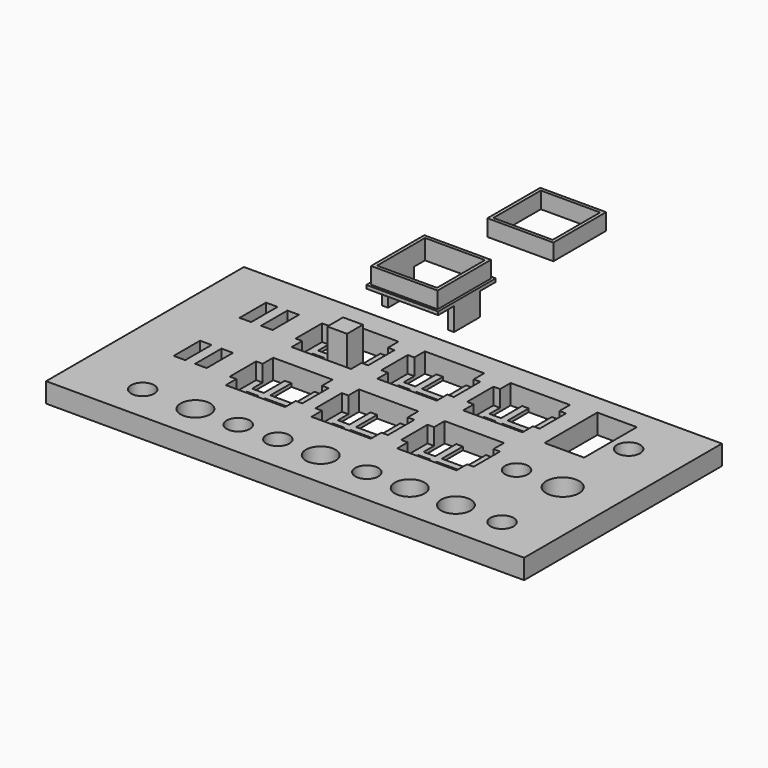
from build123d import *

# Parameters (mm, degrees)
F0_W      = 145
F0_H      = 75
F0_R      = 3.5
F0_R_2    = 4.5
F0_R_3    = 5
F0_W_2    = 12
F0_H_2    = 20
F0_W_3    = 3
F0_H_3    = 10
F1_DEPTH  = 1
F2_DEPTH  = 5
F3_W      = 18
F3_H      = 18
F4_DEPTH  = 5
F5_W      = 2
F5_H      = 10
F6_DEPTH  = 5
F8_DEPTH  = 5
F7_W      = 1.8
F7_H      = 9.8
F9_DEPTH  = 1
F10_DEPTH = 6.95
F11_W     = 20.2
F11_H     = 20.2
F11_W_2   = 18.2
F11_H_2   = 18.2
F12_DEPTH = 5
F13_W     = 6
F13_H     = 2
F14_DEPTH = 10


with BuildPart() as f1:
    # F0 (on Top) → F1 (new body)
    with BuildSketch(Plane.XY):
        with Locations((-82.504784634, -17.5405644029)):
            Rectangle(F0_W, F0_H)
        with Locations((-134.504784634, -44.0405644029)):
            Circle(F0_R, mode=Mode.SUBTRACT)
        with Locations((-118.504784634, -44.0405644029)):
            Circle(F0_R_2, mode=Mode.SUBTRACT)
        with Locations((-105.504784634, -44.0405644029)):
            Circle(F0_R, mode=Mode.SUBTRACT)
        with Locations((-93.504784634, -44.0405644029)):
            Circle(F0_R, mode=Mode.SUBTRACT)
        Polygon((-129.504784634, -16.0405644029), (-129.504784634, -26.0405644029), (-133.004784634, -26.0405644029), (-136.004784634, -26.0405644029), (-139.504784634, -26.0405644029), (-139.504784634, -16.0405644029), (-136.004784634, -16.0405644029), (-133.004784634, -16.0405644029), align=None, mode=Mode.SUBTRACT)
        Polygon((-102.504784634, -22.0405644029), (-102.504784634, -30.0405644029), (-105.9770819313, -30.0405644029), (-107.9770819313, -30.0405644029), (-114.9770819313, -30.0405644029), (-116.9770819313, -30.0405644029), (-120.504784634, -30.0405644029), (-120.504784634, -22.0405644029), (-120.504784634, -20.0405644029), (-120.504784634, -12.0405644029), (-116.9770819313, -12.0405644029), (-114.9770819313, -12.0405644029), (-107.9770819313, -12.0405644029), (-105.9770819313, -12.0405644029), (-102.504784634, -12.0405644029), (-102.504784634, -20.0405644029), align=None, mode=Mode.SUBTRACT)
        Polygon((-76.504784634, -12.0405644029), (-76.504784634, -20.0405644029), (-76.504784634, -22.0405644029), (-76.504784634, -30.0405644029), (-79.9770819313, -30.0405644029), (-81.9770819313, -30.0405644029), (-88.9770819313, -30.0405644029), (-90.9770819313, -30.0405644029), (-94.504784634, -30.0405644029), (-94.504784634, -22.0405644029), (-94.504784634, -20.0405644029), (-94.504784634, -12.0405644029), (-90.9770819313, -12.0405644029), (-88.9770819313, -12.0405644029), (-81.9770819313, -12.0405644029), (-79.9770819313, -12.0405644029), align=None, mode=Mode.SUBTRACT)
        with Locations((-80.504784634, -44.0405644029)):
            Circle(F0_R_2, mode=Mode.SUBTRACT)
        with Locations((-66.504784634, -44.0405644029)):
            Circle(F0_R, mode=Mode.SUBTRACT)
        with Locations((-53.504784634, -44.0405644029)):
            Circle(F0_R_2, mode=Mode.SUBTRACT)
        with Locations((-39.504784634, -44.0405644029)):
            Circle(F0_R_2, mode=Mode.SUBTRACT)
        with Locations((-25.504784634, -44.0405644029)):
            Circle(F0_R, mode=Mode.SUBTRACT)
        Polygon((-50.504784634, -12.0405644029), (-50.504784634, -20.0405644029), (-50.504784634, -22.0405644029), (-50.504784634, -30.0405644029), (-53.9770819313, -30.0405644029), (-55.9770819313, -30.0405644029), (-62.9770819313, -30.0405644029), (-64.9770819313, -30.0405644029), (-68.504784634, -30.0405644029), (-68.504784634, -22.0405644029), (-68.504784634, -20.0405644029), (-68.504784634, -12.0405644029), (-64.9770819313, -12.0405644029), (-62.9770819313, -12.0405644029), (-55.9770819313, -12.0405644029), (-53.9770819313, -12.0405644029), align=None, mode=Mode.SUBTRACT)
        with Locations((-39.504784634, -21.0405644029)):
            Circle(F0_R, mode=Mode.SUBTRACT)
        with Locations((-25.504784634, -21.0405644029)):
            Circle(F0_R_3, mode=Mode.SUBTRACT)
        Polygon((-129.504784634, 8.9594355971), (-129.504784634, -1.0405644029), (-133.004784634, -1.0405644029), (-136.004784634, -1.0405644029), (-139.504784634, -1.0405644029), (-139.504784634, 8.9594355971), (-136.004784634, 8.9594355971), (-133.004784634, 8.9594355971), align=None, mode=Mode.SUBTRACT)
        Polygon((-102.504784634, 2.9594355971), (-102.504784634, -5.0405644029), (-106.004784634, -5.0405644029), (-108.004784634, -5.0405644029), (-115.004784634, -5.0405644029), (-117.004784634, -5.0405644029), (-120.504784634, -5.0405644029), (-120.504784634, 2.9594355971), (-120.504784634, 4.9594355971), (-120.504784634, 12.9594355971), (-117.004784634, 12.9594355971), (-115.004784634, 12.9594355971), (-108.004784634, 12.9594355971), (-106.004784634, 12.9594355971), (-102.504784634, 12.9594355971), (-102.504784634, 4.9594355971), align=None, mode=Mode.SUBTRACT)
        Polygon((-94.504784634, 12.9594355971), (-91.004784634, 12.9594355971), (-89.004784634, 12.9594355971), (-82.004784634, 12.9594355971), (-80.004784634, 12.9594355971), (-76.504784634, 12.9594355971), (-76.504784634, 4.9594355971), (-76.504784634, 2.9594355971), (-76.504784634, -5.0405644029), (-80.004784634, -5.0405644029), (-82.004784634, -5.0405644029), (-89.004784634, -5.0405644029), (-91.004784634, -5.0405644029), (-94.504784634, -5.0405644029), (-94.504784634, 2.9594355971), (-94.504784634, 4.9594355971), align=None, mode=Mode.SUBTRACT)
        Polygon((-68.504784634, 12.9594355971), (-65.004784634, 12.9594355971), (-63.004784634, 12.9594355971), (-56.004784634, 12.9594355971), (-54.004784634, 12.9594355971), (-50.504784634, 12.9594355971), (-50.504784634, 4.9594355971), (-50.504784634, 2.9594355971), (-50.504784634, -5.0405644029), (-54.004784634, -5.0405644029), (-56.004784634, -5.0405644029), (-63.004784634, -5.0405644029), (-65.004784634, -5.0405644029), (-68.504784634, -5.0405644029), (-68.504784634, 2.9594355971), (-68.504784634, 4.9594355971), align=None, mode=Mode.SUBTRACT)
        with Locations((-37.004784634, 3.9594355971)):
            Rectangle(F0_W_2, F0_H_2, mode=Mode.SUBTRACT)
        with Locations((-25.504784634, 3.9594355971)):
            Circle(F0_R, mode=Mode.SUBTRACT)
        Polygon((-108.004784634, -5.0405644029), (-106.004784634, -5.0405644029), (-106.004784634, 2.9594355971), (-102.504784634, 2.9594355971), (-102.504784634, 4.9594355971), (-106.004784634, 4.9594355971), (-106.004784634, 12.9594355971), (-108.004784634, 12.9594355971), (-108.004784634, 4.9594355971), (-115.004784634, 4.9594355971), (-115.004784634, 12.9594355971), (-117.004784634, 12.9594355971), (-117.004784634, 4.9594355971), (-120.504784634, 4.9594355971), (-120.504784634, 2.9594355971), (-117.004784634, 2.9594355971), (-117.004784634, -5.0405644029), (-115.004784634, -5.0405644029), (-115.004784634, 2.9594355971), (-108.004784634, 2.9594355971), align=None)
        Polygon((-107.9770819313, -30.0405644029), (-105.9770819313, -30.0405644029), (-105.9770819313, -22.0405644029), (-102.504784634, -22.0405644029), (-102.504784634, -20.0405644029), (-105.9770819313, -20.0405644029), (-105.9770819313, -12.0405644029), (-107.9770819313, -12.0405644029), (-107.9770819313, -20.0405644029), (-114.9770819313, -20.0405644029), (-114.9770819313, -12.0405644029), (-116.9770819313, -12.0405644029), (-116.9770819313, -20.0405644029), (-120.504784634, -20.0405644029), (-120.504784634, -22.0405644029), (-116.9770819313, -22.0405644029), (-116.9770819313, -30.0405644029), (-114.9770819313, -30.0405644029), (-114.9770819313, -22.0405644029), (-107.9770819313, -22.0405644029), align=None)
        Polygon((-91.004784634, 12.9594355971), (-91.004784634, 4.9594355971), (-94.504784634, 4.9594355971), (-94.504784634, 2.9594355971), (-91.004784634, 2.9594355971), (-91.004784634, -5.0405644029), (-89.004784634, -5.0405644029), (-89.004784634, 2.9594355971), (-82.004784634, 2.9594355971), (-82.004784634, -5.0405644029), (-80.004784634, -5.0405644029), (-80.004784634, 2.9594355971), (-76.504784634, 2.9594355971), (-76.504784634, 4.9594355971), (-80.004784634, 4.9594355971), (-80.004784634, 12.9594355971), (-82.004784634, 12.9594355971), (-82.004784634, 4.9594355971), (-89.004784634, 4.9594355971), (-89.004784634, 12.9594355971), align=None)
        Polygon((-65.004784634, 12.9594355971), (-65.004784634, 4.9594355971), (-68.504784634, 4.9594355971), (-68.504784634, 2.9594355971), (-65.004784634, 2.9594355971), (-65.004784634, -5.0405644029), (-63.004784634, -5.0405644029), (-63.004784634, 2.9594355971), (-56.004784634, 2.9594355971), (-56.004784634, -5.0405644029), (-54.004784634, -5.0405644029), (-54.004784634, 2.9594355971), (-50.504784634, 2.9594355971), (-50.504784634, 4.9594355971), (-54.004784634, 4.9594355971), (-54.004784634, 12.9594355971), (-56.004784634, 12.9594355971), (-56.004784634, 4.9594355971), (-63.004784634, 4.9594355971), (-63.004784634, 12.9594355971), align=None)
        Polygon((-50.504784634, -22.0405644029), (-50.504784634, -20.0405644029), (-53.9770819313, -20.0405644029), (-53.9770819313, -12.0405644029), (-55.9770819313, -12.0405644029), (-55.9770819313, -20.0405644029), (-62.9770819313, -20.0405644029), (-62.9770819313, -12.0405644029), (-64.9770819313, -12.0405644029), (-64.9770819313, -20.0405644029), (-68.504784634, -20.0405644029), (-68.504784634, -22.0405644029), (-64.9770819313, -22.0405644029), (-64.9770819313, -30.0405644029), (-62.9770819313, -30.0405644029), (-62.9770819313, -22.0405644029), (-55.9770819313, -22.0405644029), (-55.9770819313, -30.0405644029), (-53.9770819313, -30.0405644029), (-53.9770819313, -22.0405644029), align=None)
        Polygon((-76.504784634, -22.0405644029), (-76.504784634, -20.0405644029), (-79.9770819313, -20.0405644029), (-79.9770819313, -12.0405644029), (-81.9770819313, -12.0405644029), (-81.9770819313, -20.0405644029), (-88.9770819313, -20.0405644029), (-88.9770819313, -12.0405644029), (-90.9770819313, -12.0405644029), (-90.9770819313, -20.0405644029), (-94.504784634, -20.0405644029), (-94.504784634, -22.0405644029), (-90.9770819313, -22.0405644029), (-90.9770819313, -30.0405644029), (-88.9770819313, -30.0405644029), (-88.9770819313, -22.0405644029), (-81.9770819313, -22.0405644029), (-81.9770819313, -30.0405644029), (-79.9770819313, -30.0405644029), (-79.9770819313, -22.0405644029), align=None)
        with Locations((-134.504784634, 3.9594355971)):
            Rectangle(F0_W_3, F0_H_3)
        with Locations((-134.504784634, -21.0405644029)):
            Rectangle(F0_W_3, F0_H_3)
    extrude(amount=F1_DEPTH)

    # F2 (add): a face of the model
    f2_faces = [f1.faces().sort_by_distance(p)[0] for p in [
        (-82.504784634, 18.3269528253, 1),
    ]]
    extrude(f2_faces, amount=F2_DEPTH)

    # F3 (on face) → F4 (cut)
    with BuildSketch(Plane.XY.offset(6)):
        with Locations((-111.504784634, 3.9594355971)):
            Rectangle(F3_W, F3_H)
        with Locations((-111.504784634, -21.0405644029)):
            Rectangle(F3_W, F3_H)
        with Locations((-85.504784634, 3.9594355971)):
            Rectangle(F3_W, F3_H)
        with Locations((-85.504784634, -21.0405644029)):
            Rectangle(F3_W, F3_H)
        with Locations((-59.504784634, 3.9594355971)):
            Rectangle(F3_W, F3_H)
        with Locations((-59.504784634, -21.0405644029)):
            Rectangle(F3_W, F3_H)
    extrude(amount=-F4_DEPTH, mode=Mode.SUBTRACT)

    # F5 (on face) → F6 (cut)
    with BuildSketch(Plane.XY.offset(6)):
        with Locations((-121.504784634, 3.9594355971)):
            Rectangle(F5_W, F5_H)
        with Locations((-101.504784634, 3.9594355971)):
            Rectangle(F5_W, F5_H)
        with Locations((-75.504784634, 3.9594355971)):
            Rectangle(F5_W, F5_H)
        with Locations((-95.504784634, 3.9594355971)):
            Rectangle(F5_W, F5_H)
        with Locations((-49.504784634, 3.9594355971)):
            Rectangle(F5_W, F5_H)
        with Locations((-69.504784634, 3.9594355971)):
            Rectangle(F5_W, F5_H)
        with Locations((-121.504784634, -21.0405644029)):
            Rectangle(F5_W, F5_H)
        with Locations((-101.504784634, -21.0405644029)):
            Rectangle(F5_W, F5_H)
        with Locations((-95.504784634, -21.0405644029)):
            Rectangle(F5_W, F5_H)
        with Locations((-75.504784634, -21.0405644029)):
            Rectangle(F5_W, F5_H)
        with Locations((-69.504784634, -21.0405644029)):
            Rectangle(F5_W, F5_H)
        with Locations((-49.504784634, -21.0405644029)):
            Rectangle(F5_W, F5_H)
    extrude(amount=-F6_DEPTH, mode=Mode.SUBTRACT)

    # F13 (on face) → F14 (join)
    with BuildSketch(Plane.XY.offset(1)):
        with Locations((-111.504784634, 5.9594355971)):
            Rectangle(F13_W, F13_H)
        with Locations((-111.504784634, 3.9594355971)):
            Rectangle(F13_W, F13_H)
        with Locations((-111.504784634, 1.9594355971)):
            Rectangle(F13_W, F13_H)
    extrude(amount=F14_DEPTH)


with BuildPart() as f8:
    # F7 (on Top) → F8 (new body)
    with BuildSketch(Plane.XY):
        Polygon((-107.7882362008, 82.0260888338), (-106.7882362008, 82.0260888338), (-106.7882362008, 92.0260888338), (-107.7882362008, 92.0260888338), (-107.7882362008, 87.5260888338), (-107.7882362008, 86.5260888338), align=None)
        Polygon((-107.7882362008, 92.0260888338), (-106.7882362008, 92.0260888338), (-106.7882362008, 97.0260888338), (-126.7882362008, 97.0260888338), (-126.7882362008, 92.0260888338), (-125.7882362008, 92.0260888338), (-125.7882362008, 96.0260888338), (-107.7882362008, 96.0260888338), align=None)
        Polygon((-126.7882362008, 77.0260888338), (-106.7882362008, 77.0260888338), (-106.7882362008, 82.0260888338), (-107.7882362008, 82.0260888338), (-107.7882362008, 78.0260888338), (-125.7882362008, 78.0260888338), (-125.7882362008, 82.0260888338), (-126.7882362008, 82.0260888338), align=None)
        Polygon((-126.7882362008, 92.0260888338), (-126.7882362008, 82.0260888338), (-125.7882362008, 82.0260888338), (-125.7882362008, 86.5260888338), (-125.7882362008, 87.5260888338), (-125.7882362008, 92.0260888338), align=None)
    extrude(amount=F8_DEPTH)


with BuildPart() as f9:
    # F7 (on Top) → F9 (new body)
    with BuildSketch(Plane.XY):
        Polygon((-132.6183355093, 38.3936729491), (-110.8183355093, 38.3936729491), (-110.8183355093, 44.3936729491), (-112.6183355093, 44.3936729491), (-112.6183355093, 40.1936729491), (-130.8183355093, 40.1936729491), (-130.8183355093, 44.3936729491), (-132.6183355093, 44.3936729491), align=None)
        with Locations((-111.7183355093, 49.2936729491)):
            Rectangle(F7_W, F7_H)
        with Locations((-131.7183355093, 49.2936729491)):
            Rectangle(F7_W, F7_H)
        Polygon((-112.6183355093, 54.1936729491), (-110.8183355093, 54.1936729491), (-110.8183355093, 60.1936729491), (-132.6183355093, 60.1936729491), (-132.6183355093, 54.1936729491), (-130.8183355093, 54.1936729491), (-130.8183355093, 58.3936729491), (-112.6183355093, 58.3936729491), align=None)
    extrude(amount=F9_DEPTH)

    # F7 (on Top) → F10 (join)
    with BuildSketch(Plane.XY):
        with Locations((-131.7183355093, 49.2936729491)):
            Rectangle(F7_W, F7_H)
        with Locations((-111.7183355093, 49.2936729491)):
            Rectangle(F7_W, F7_H)
    extrude(amount=-F10_DEPTH)

    # F11 (on face) → F12 (join)
    with BuildSketch(Plane.XY.offset(1)):
        with Locations((-121.7183355093, 49.2936729491)):
            Rectangle(F11_W, F11_H)
        with Locations((-121.7183355093, 49.2936729491)):
            Rectangle(F11_W_2, F11_H_2, mode=Mode.SUBTRACT)
    extrude(amount=F12_DEPTH)


solid = Compound([f1.part, f8.part, f9.part])
